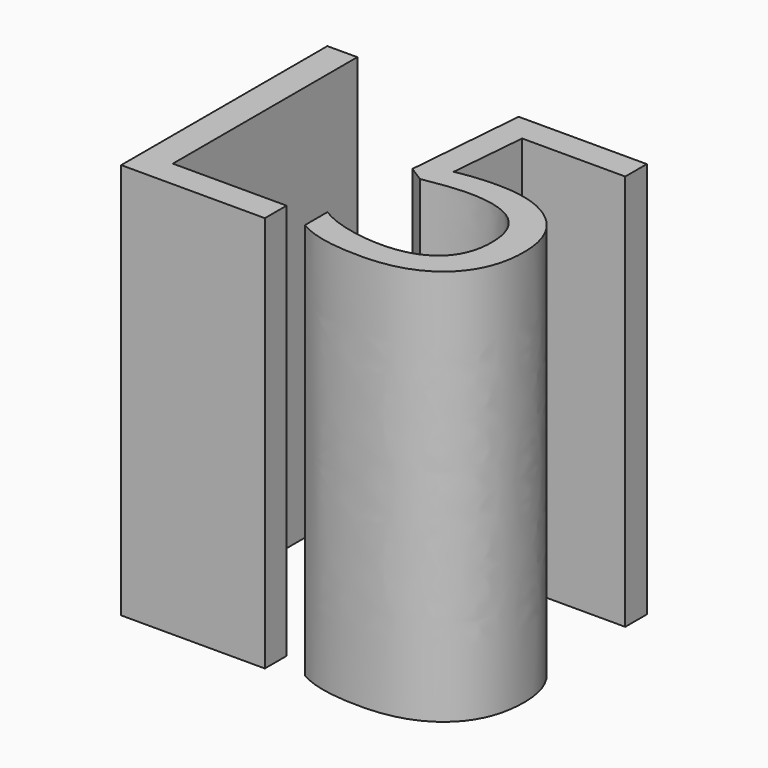
from build123d import *

# Parameters (mm, degrees)
F0_TEXT_SIZE = 9.1064314172
F1_DEPTH     = 10


# Not quite as in the source:
# - Text() gives the source's letters only with a copy of the font that has no kerning and outlines rounded to 1/6400 em; it was checked with that copy


with BuildPart() as f1:
    # F0 (on Top) → F1 (new body)
    with BuildSketch(Plane.XY):
        with Locations((-5, -3.2783153102)):
            Text('L5', F0_TEXT_SIZE, font='Open Sans', text_align=(TextAlign.LEFT, TextAlign.BOTTOM))
    extrude(amount=F1_DEPTH)


solid = f1.part
